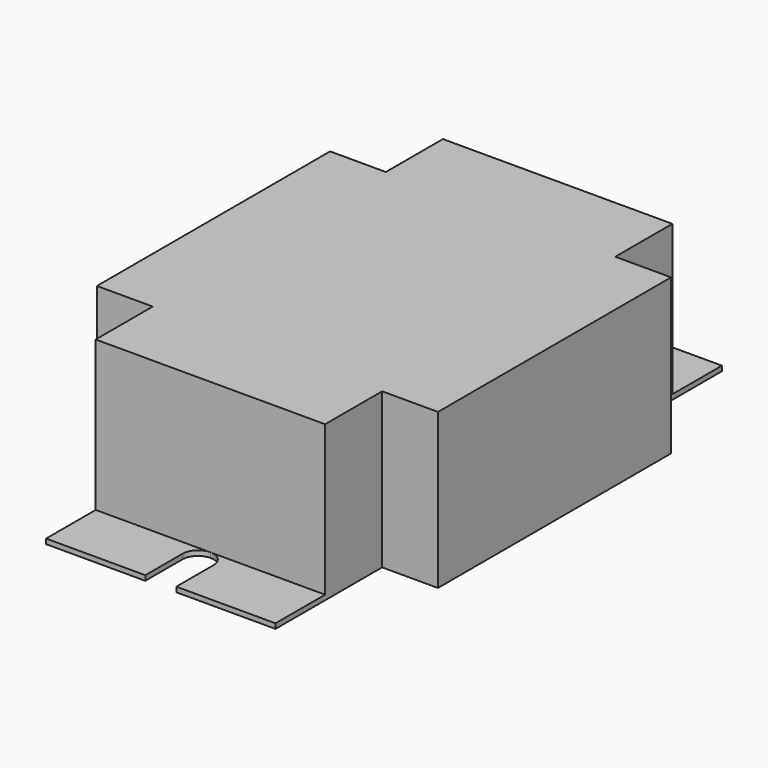
from build123d import *

# Parameters (mm, degrees)
F1_DEPTH    = 25
F2_W        = 37
F2_H        = 0.8
F3_DEPTH    = 10
F4_W        = 37
F4_H        = 0.8
F5_DEPTH    = 10
F6_T        = 0.8
F6_T3_DEPTH = 26.6
F6_T5_DEPTH = 38.6
F9_DEPTH    = 2


# Not quite as in the source:
# - a shell that OpenCascade refuses in one call is made with other operations: the cavity is built on its own and cut out


with BuildPart() as f1:
    # F0 (on Top) → F1 (new body)
    with BuildSketch(Plane.XY):
        Polygon((-33.6095448622, 23.5), (-33.6095448622, -23.5), (-24.6095448622, -23.5), (-24.6095448622, -35), (12.3904551378, -35), (12.3904551378, -23.5), (21.3904551378, -23.5), (21.3904551378, 23.5), (12.3904551378, 23.5), (12.3904551378, 35), (-24.6095448622, 35), (-24.6095448622, 23.5), align=None)
    extrude(amount=F1_DEPTH)

    # F2 (on face) → F3 (join)
    with BuildSketch(Plane.XZ.offset(35)):
        with Locations((-6.1095448622, 0.4)):
            Rectangle(F2_W, F2_H)
    extrude(amount=F3_DEPTH)

    # F4 (on face) → F5 (join)
    with BuildSketch(Plane(origin=(0, 35, 0), x_dir=(-1, 0, 0), z_dir=(0, 1, 0))):
        with Locations((6.1095448622, 0.4)):
            Rectangle(F4_W, F4_H)
    extrude(amount=F5_DEPTH)

    # F6: shell of thickness 0.8, made by hand


with BuildPart() as f6_core1:
    # F6_t2: copy of F1
    add(f1.part)

    # the walls: a layer under each face that stays
    f6_faces = [f6_core1.faces().sort_by_distance(p)[0] for p in [
        (-33.6095448622, 0, 12.5),
        (-6.1095448622, 0, 25),
        (-24.6095448622, 34.25, 12.5),
        (-6.1095448622, 40, 0.8),
        (-6.1095448622, 45, 0.4),
        (-6.1095448622, 35, 12.9),
        (12.3904551378, 34.25, 12.5),
        (16.8904551378, 23.5, 12.5),
        (21.3904551378, 0, 12.5),
        (16.8904551378, -23.5, 12.5),
        (12.3904551378, -34.25, 12.5),
        (-6.1095448622, -40, 0.8),
        (-6.1095448622, -45, 0.4),
        (-6.1095448622, -35, 12.9),
        (-24.6095448622, -34.25, 12.5),
        (-29.1095448622, -23.5, 12.5),
        (-29.1095448622, 23.5, 12.5),
    ]]
    thicken(f6_faces, amount=-F6_T, mode=Mode.SUBTRACT)

    # F6_s4 → F6_t3 (cut)
    with BuildSketch(Plane.XY.offset(-0.8)):
        Polygon((-24.6175448622, 23.508), (-23.8095448622, 23.5), (-23.8095448622, 22.7), (-24.6095448622, 22.7), align=None)
        Polygon((12.3984551378, 23.508), (11.5904551378, 23.5), (11.5904551378, 22.7), (12.3904551378, 22.7), align=None)
        Polygon((12.3984551378, -23.508), (12.3904551378, -22.7), (11.5904551378, -22.7), (11.5904551378, -23.5), align=None)
        Polygon((-24.6175448622, -23.508), (-23.8095448622, -23.5), (-23.8095448622, -22.7), (-24.6095448622, -22.7), align=None)
    extrude(amount=F6_T3_DEPTH, mode=Mode.SUBTRACT)

    # F6_s6 → F6_t5 (cut)
    with BuildSketch(Plane.YZ.offset(-25.4095448622)):
        Polygon((35.008, 0.808), (35, 0), (34.2, 0), (34.2, 0.8), align=None)
        Polygon((-35.008, 0.808), (-35, 0), (-34.2, 0), (-34.2, 0.8), align=None)
    extrude(amount=F6_T5_DEPTH, mode=Mode.SUBTRACT)


with BuildPart() as f1_1:
    add(f1.part)

    # what is left inside the walls is the cavity
    f6_cavity = [f6_core1.part.solids().sort_by_distance(p)[0] for p in [
        (-6.109545, -11.4, 24.192),
    ]]
    add(f6_cavity, mode=Mode.SUBTRACT)

    # F8 (on face) + F7 (on face) → F9 (cut)
    with BuildSketch(Plane.XY.offset(0.8)):
        with BuildLine():
            Line((-8.6095448622, -37.5000002948), (-8.6095448622, -45))
            Line((-8.6095448622, -45), (-3.6095448622, -45))
            Line((-3.6095448622, -45), (-3.6095448622, -37.5))
            ThreePointArc((-3.6095448622, -37.5), (-4.3417779216, -35.7322330347), (-6.1095448972, -35))
            ThreePointArc((-6.1095448972, -35), (-7.8773119318, -35.7322331636), (-8.6095448622, -37.5000002948))
        make_face()
    with BuildSketch(Plane.XY.offset(0.8)):
        with BuildLine():
            Line((-3.6095448622, 37.5), (-3.6095448622, 45))
            Line((-3.6095448622, 45), (-8.6095448622, 45))
            Line((-8.6095448622, 45), (-8.6095448622, 37.5))
            ThreePointArc((-8.6095448622, 37.5), (-7.8773118305, 35.7322330623), (-6.1095449054, 35))
            ThreePointArc((-6.1095449054, 35), (-4.3417779245, 35.7322330318), (-3.6095448622, 37.5))
        make_face()
    extrude(amount=-F9_DEPTH, mode=Mode.SUBTRACT)


solid = f1_1.part
